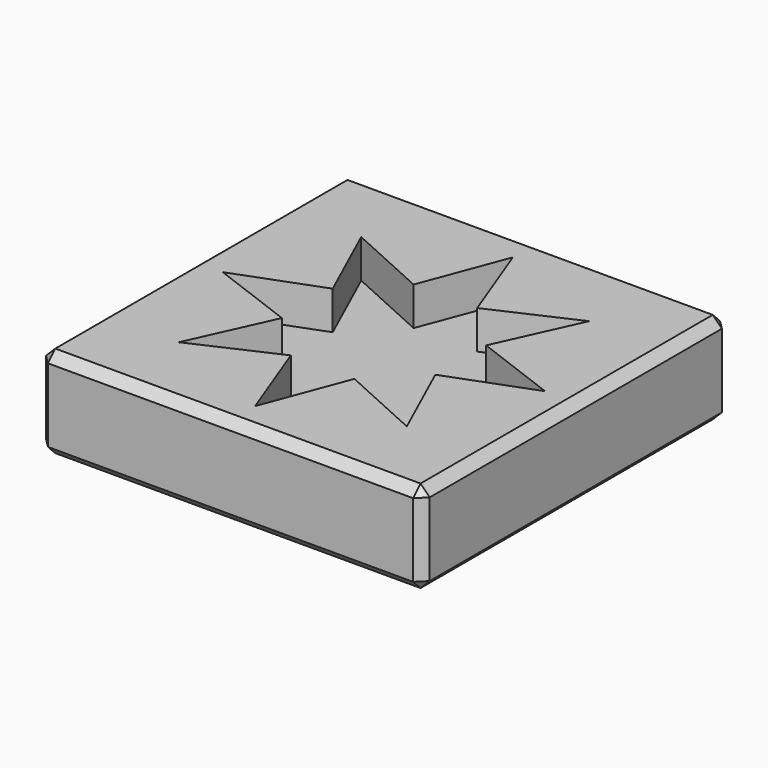
from build123d import *

# Parameters (mm, degrees)
F0_W     = 25
F0_H     = 25
F1_DEPTH = 6
F2_W     = 21
F2_H     = 21
F2_W_2   = 11
F2_H_2   = 11
F2_W_3   = 5
F2_H_3   = 5
F3_DEPTH = 2.7
F4_START = 3.5
F4_DEPTH = 2.501
F5_SIZE  = 0.6
F6_SIZE2 = 2.69999
F6_SIZE  = 0.99999


# Not quite as in the source:
# - a fillet or chamfer is up to 0.001 mm smaller than in the source, because OpenCascade refuses the exact size


with BuildPart() as f1:
    # F0 (on Top) → F1 (new body)
    with BuildSketch(Plane.XY):
        Rectangle(F0_W, F0_H)
        Polygon((-7.4246212025, 7.4246212025), (-2.0710678119, 5), (0, 10.5), (2.0710678119, 5), (7.4246212025, 7.4246212025), (5, 2.0710678119), (10.5, 0), (5, -2.0710678119), (7.4246212025, -7.4246212025), (2.0710678119, -5), (0, -10.5), (-2.0710678119, -5), (-7.4246212025, -7.4246212025), (-5, -2.0710678119), (-10.5, 0), (-5, 2.0710678119), align=None, mode=Mode.SUBTRACT)
        Polygon((0, 10.5), (-2.0710678119, 5), (-7.4246212025, 7.4246212025), (-5, 2.0710678119), (-10.5, 0), (-5, -2.0710678119), (-7.4246212025, -7.4246212025), (-2.0710678119, -5), (0, -10.5), (2.0710678119, -5), (7.4246212025, -7.4246212025), (5, -2.0710678119), (10.5, 0), (5, 2.0710678119), (7.4246212025, 7.4246212025), (2.0710678119, 5), align=None)
    extrude(amount=F1_DEPTH)

    # F2 (on Top) → F3 (cut)
    with BuildSketch(Plane.XY):
        Rectangle(F2_W, F2_H)
        Rectangle(F2_W_2, F2_H_2, mode=Mode.SUBTRACT)
        Rectangle(F2_W_3, F2_H_3)
    extrude(amount=F3_DEPTH, mode=Mode.SUBTRACT)

    # F0 (on Top) → F4 (cut)
    with BuildSketch(Plane.XY.offset(F4_START)):
        Polygon((0, 10.5), (-2.0710678119, 5), (-7.4246212025, 7.4246212025), (-5, 2.0710678119), (-10.5, 0), (-5, -2.0710678119), (-7.4246212025, -7.4246212025), (-2.0710678119, -5), (0, -10.5), (2.0710678119, -5), (7.4246212025, -7.4246212025), (5, -2.0710678119), (10.5, 0), (5, 2.0710678119), (7.4246212025, 7.4246212025), (2.0710678119, 5), align=None)
    extrude(amount=F4_DEPTH, mode=Mode.SUBTRACT)

    # F5
    f5_edges = [f1.edges().sort_by_distance(p)[0] for p in [
        (0, -12.5, 6),
        (-12.5, -12.5, 3),
        (-12.5, 0, 6),
        (-12.5, 12.5, 3),
        (0, 12.5, 6),
        (12.5, 0, 6),
        (12.5, -12.5, 3),
        (12.5, 12.5, 3),
        (0, -12.5, 0),
        (12.5, 0, 0),
        (0, 12.5, 0),
        (-12.5, 0, 0),
    ]]
    chamfer(f5_edges, length=F5_SIZE)

    # F6 (size 1 and 2.7 in the source; OpenCascade refuses exactly that, so slightly less here)
    f6_edges = [f1.edges().sort_by_distance(p)[0] for p in [
        (-5.5, 0, 0),
        (0, 5.5, 0),
        (5.5, 0, 0),
        (0, -5.5, 0),
        (-2.5, 0, 0),
        (0, -2.5, 0),
        (2.5, 0, 0),
        (0, 2.5, 0),
    ]]
    f6_side = f1.faces().sort_by_distance((-5.344437, 0, 0))[0]
    chamfer(f6_edges, length=F6_SIZE, length2=F6_SIZE2, reference=f6_side)


solid = f1.part
